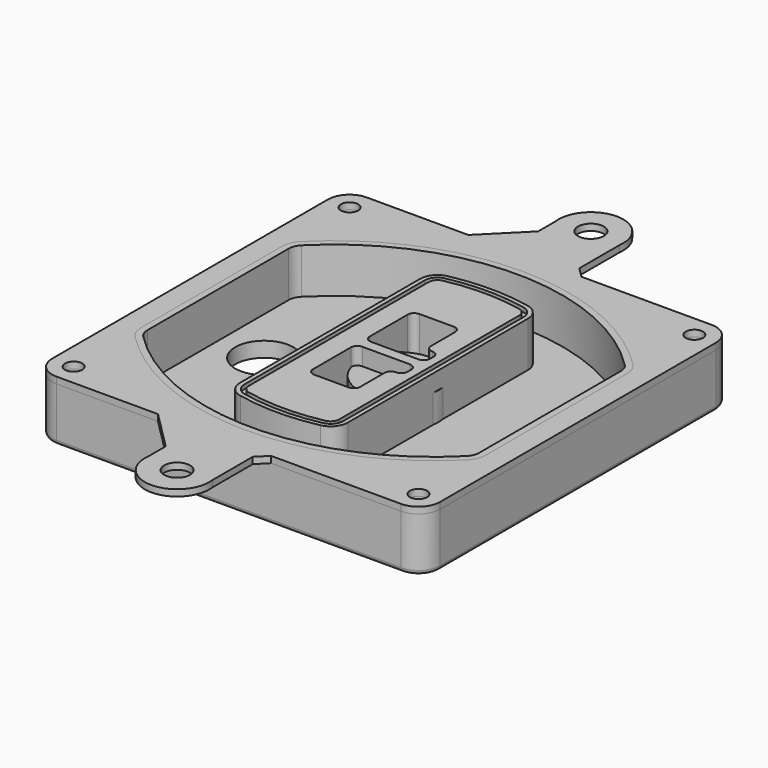
from build123d import *

# Parameters (mm, degrees)
F0_R      = 4
F1_DEPTH  = 25
F2_DEPTH  = 3
F3_DEPTH  = 18
F5_DEPTH  = 21
F6_DEPTH  = 2
F8_DEPTH  = 20
F9_DEPTH  = 16
F10_DEPTH = 25
F7_R      = 6
F7_R_2    = 4
F11_DEPTH = 6
F13_DEPTH = 9
F15_R     = 2
F16_R     = 6
F16_R_2   = 4
F17_DEPTH = 3


# Not quite as in the source:
# - a feature of the source that left no trace in its solid (it failed there, or was rolled back) is left out
# - a feature names something its author has since deleted; it is built from what else it names


with BuildPart() as f1:
    # F0 (on Top) → F1 (new body)
    with BuildSketch(Plane.XY):
        with BuildLine():
            ThreePointArc((-90, -80), (-87.0710678119, -87.0710678119), (-80, -90))
            Line((-80, -90), (80, -90))
            ThreePointArc((80, -90), (87.0710678119, -87.0710678119), (90, -80))
            Line((90, -80), (90, 80))
            ThreePointArc((90, 80), (87.0710678119, 87.0710678119), (80, 90))
            Line((80, 90), (-80, 90))
            ThreePointArc((-80, 90), (-87.0710678119, 87.0710678119), (-90, 80))
            Line((-90, 80), (-90, -80))
        make_face()
        with Locations((-80, -80)):
            Circle(F0_R, mode=Mode.SUBTRACT)
        with Locations((80, -80)):
            Circle(F0_R, mode=Mode.SUBTRACT)
        with Locations((-80, 80)):
            Circle(F0_R, mode=Mode.SUBTRACT)
        with BuildLine():
            ThreePointArc((-84, 40.977524478), (-82.9361107095, 46.3307515151), (-79.9061371841, 50.8703727074))
            ThreePointArc((-79.9061371841, 50.8703727074), (0, 84), (79.9061371841, 50.8703727074))
            ThreePointArc((79.9061371841, 50.8703727074), (82.9361107095, 46.3307515151), (84, 40.977524478))
            Line((84, 40.977524478), (84, -40.977524478))
            ThreePointArc((84, -40.977524478), (82.9361107095, -46.3307515151), (79.9061371841, -50.8703727074))
            ThreePointArc((79.9061371841, -50.8703727074), (0, -84), (-79.9061371841, -50.8703727074))
            ThreePointArc((-79.9061371841, -50.8703727074), (-82.9361107095, -46.3307515151), (-84, -40.977524478))
            Line((-84, -40.977524478), (-84, 40.977524478))
        make_face(mode=Mode.SUBTRACT)
        with Locations((80, 80)):
            Circle(F0_R, mode=Mode.SUBTRACT)
        with BuildLine():
            ThreePointArc((79.9061371841, 50.8703727074), (0, 84), (-79.9061371841, 50.8703727074))
            ThreePointArc((-79.9061371841, 50.8703727074), (-82.9361107095, 46.3307515151), (-84, 40.977524478))
            Line((-84, 40.977524478), (-84, -40.977524478))
            ThreePointArc((-84, -40.977524478), (-82.9361107095, -46.3307515151), (-79.9061371841, -50.8703727074))
            ThreePointArc((-79.9061371841, -50.8703727074), (0, -84), (79.9061371841, -50.8703727074))
            ThreePointArc((79.9061371841, -50.8703727074), (82.9361107095, -46.3307515151), (84, -40.977524478))
            Line((84, -40.977524478), (84, 40.977524478))
            ThreePointArc((84, 40.977524478), (82.9361107095, 46.3307515151), (79.9061371841, 50.8703727074))
        make_face()
        with BuildLine():
            Line((-80, -40.977524478), (-80, 40.977524478))
            ThreePointArc((-80, 40.977524478), (-79.2400790782, 44.801258076), (-77.0758122744, 48.0438446418))
            ThreePointArc((-77.0758122744, 48.0438446418), (0, 80), (77.0758122744, 48.0438446418))
            ThreePointArc((77.0758122744, 48.0438446418), (79.2400790782, 44.801258076), (80, 40.977524478))
            Line((80, 40.977524478), (80, -40.977524478))
            ThreePointArc((80, -40.977524478), (79.2400790782, -44.801258076), (77.0758122744, -48.0438446418))
            ThreePointArc((77.0758122744, -48.0438446418), (0, -80), (-77.0758122744, -48.0438446418))
            ThreePointArc((-77.0758122744, -48.0438446418), (-79.2400790782, -44.801258076), (-80, -40.977524478))
        make_face(mode=Mode.SUBTRACT)
        with BuildLine():
            ThreePointArc((-77.0758122744, 48.0438446418), (-79.2400790782, 44.801258076), (-80, 40.977524478))
            Line((-80, 40.977524478), (-80, -40.977524478))
            ThreePointArc((-80, -40.977524478), (-79.2400790782, -44.801258076), (-77.0758122744, -48.0438446418))
            ThreePointArc((-77.0758122744, -48.0438446418), (0, -80), (77.0758122744, -48.0438446418))
            ThreePointArc((77.0758122744, -48.0438446418), (79.2400790782, -44.801258076), (80, -40.977524478))
            Line((80, -40.977524478), (80, 40.977524478))
            ThreePointArc((80, 40.977524478), (79.2400790782, 44.801258076), (77.0758122744, 48.0438446418))
            ThreePointArc((77.0758122744, 48.0438446418), (0, 80), (-77.0758122744, 48.0438446418))
        make_face()
        with BuildLine():
            ThreePointArc((74.9530685921, 45.9239485927), (76.4680553548, 43.6541379966), (77, 40.977524478))
            Line((77, 40.977524478), (77, -40.977524478))
            ThreePointArc((77, -40.977524478), (76.4680553548, -43.6541379966), (74.9530685921, -45.9239485927))
            ThreePointArc((74.9530685921, -45.9239485927), (0, -77), (-74.9530685921, -45.9239485927))
            ThreePointArc((-74.9530685921, -45.9239485927), (-76.4680553548, -43.6541379966), (-77, -40.977524478))
            Line((-77, -40.977524478), (-77, 40.977524478))
            ThreePointArc((-77, 40.977524478), (-76.4680553548, 43.6541379966), (-74.9530685921, 45.9239485927))
            ThreePointArc((-74.9530685921, 45.9239485927), (0, 77), (74.9530685921, 45.9239485927))
        make_face(mode=Mode.SUBTRACT)
        with BuildLine():
            Line((77, -40.977524478), (77, 40.977524478))
            ThreePointArc((77, 40.977524478), (76.4680553548, 43.6541379966), (74.9530685921, 45.9239485927))
            ThreePointArc((74.9530685921, 45.9239485927), (0, 77), (-74.9530685921, 45.9239485927))
            ThreePointArc((-74.9530685921, 45.9239485927), (-76.4680553548, 43.6541379966), (-77, 40.977524478))
            Line((-77, 40.977524478), (-77, -40.977524478))
            ThreePointArc((-77, -40.977524478), (-76.4680553548, -43.6541379966), (-74.9530685921, -45.9239485927))
            ThreePointArc((-74.9530685921, -45.9239485927), (0, -77), (74.9530685921, -45.9239485927))
            ThreePointArc((74.9530685921, -45.9239485927), (76.4680553548, -43.6541379966), (77, -40.977524478))
        make_face()
    extrude(amount=-F1_DEPTH)

    # F0 (on Top) → F2 (join)
    with BuildSketch(Plane.XY):
        with BuildLine():
            ThreePointArc((-77.0758122744, 48.0438446418), (-79.2400790782, 44.801258076), (-80, 40.977524478))
            Line((-80, 40.977524478), (-80, -40.977524478))
            ThreePointArc((-80, -40.977524478), (-79.2400790782, -44.801258076), (-77.0758122744, -48.0438446418))
            ThreePointArc((-77.0758122744, -48.0438446418), (0, -80), (77.0758122744, -48.0438446418))
            ThreePointArc((77.0758122744, -48.0438446418), (79.2400790782, -44.801258076), (80, -40.977524478))
            Line((80, -40.977524478), (80, 40.977524478))
            ThreePointArc((80, 40.977524478), (79.2400790782, 44.801258076), (77.0758122744, 48.0438446418))
            ThreePointArc((77.0758122744, 48.0438446418), (0, 80), (-77.0758122744, 48.0438446418))
        make_face()
        with BuildLine():
            ThreePointArc((74.9530685921, 45.9239485927), (76.4680553548, 43.6541379966), (77, 40.977524478))
            Line((77, 40.977524478), (77, -40.977524478))
            ThreePointArc((77, -40.977524478), (76.4680553548, -43.6541379966), (74.9530685921, -45.9239485927))
            ThreePointArc((74.9530685921, -45.9239485927), (0, -77), (-74.9530685921, -45.9239485927))
            ThreePointArc((-74.9530685921, -45.9239485927), (-76.4680553548, -43.6541379966), (-77, -40.977524478))
            Line((-77, -40.977524478), (-77, 40.977524478))
            ThreePointArc((-77, 40.977524478), (-76.4680553548, 43.6541379966), (-74.9530685921, 45.9239485927))
            ThreePointArc((-74.9530685921, 45.9239485927), (0, 77), (74.9530685921, 45.9239485927))
        make_face(mode=Mode.SUBTRACT)
    extrude(amount=F2_DEPTH)

    # F0 (on Top) → F3 (cut)
    with BuildSketch(Plane.XY):
        with BuildLine():
            Line((77, -40.977524478), (77, 40.977524478))
            ThreePointArc((77, 40.977524478), (76.4680553548, 43.6541379966), (74.9530685921, 45.9239485927))
            ThreePointArc((74.9530685921, 45.9239485927), (0, 77), (-74.9530685921, 45.9239485927))
            ThreePointArc((-74.9530685921, 45.9239485927), (-76.4680553548, 43.6541379966), (-77, 40.977524478))
            Line((-77, 40.977524478), (-77, -40.977524478))
            ThreePointArc((-77, -40.977524478), (-76.4680553548, -43.6541379966), (-74.9530685921, -45.9239485927))
            ThreePointArc((-74.9530685921, -45.9239485927), (0, -77), (74.9530685921, -45.9239485927))
            ThreePointArc((74.9530685921, -45.9239485927), (76.4680553548, -43.6541379966), (77, -40.977524478))
        make_face()
    extrude(amount=-F3_DEPTH, mode=Mode.SUBTRACT)

    # F4 (on face) → F5 (join, through all)
    with BuildSketch(Plane.XY.offset(3)):
        with BuildLine():
            ThreePointArc((-25, -52.2388355719), (-23.2096587819, -57.2826573186), (-18.6399655469, -60.0689385728))
            ThreePointArc((-18.6399655469, -60.0689385728), (0, -62), (18.6399655469, -60.0689385728))
            ThreePointArc((18.6399655469, -60.0689385728), (23.2096587819, -57.2826573186), (25, -52.2388355719))
            Line((25, -52.2388355719), (25, 52.2388355719))
            ThreePointArc((25, 52.2388355719), (23.2096587819, 57.2826573186), (18.6399655469, 60.0689385728))
            ThreePointArc((18.6399655469, 60.0689385728), (0, 62), (-18.6399655469, 60.0689385728))
            ThreePointArc((-18.6399655469, 60.0689385728), (-23.2096587819, 57.2826573186), (-25, 52.2388355719))
            Line((-25, 52.2388355719), (-25, -52.2388355719))
        make_face()
        with BuildLine():
            ThreePointArc((18.2299741602, 58.1114128226), (21.6572440864, 56.0217018819), (23, 52.2388355719))
            Line((23, 52.2388355719), (23, -52.2388355719))
            ThreePointArc((23, -52.2388355719), (21.6572440864, -56.0217018819), (18.2299741602, -58.1114128226))
            ThreePointArc((18.2299741602, -58.1114128226), (0, -60), (-18.2299741602, -58.1114128226))
            ThreePointArc((-18.2299741602, -58.1114128226), (-21.6572440864, -56.0217018819), (-23, -52.2388355719))
            Line((-23, -52.2388355719), (-23, 52.2388355719))
            ThreePointArc((-23, 52.2388355719), (-21.6572440864, 56.0217018819), (-18.2299741602, 58.1114128226))
            ThreePointArc((-18.2299741602, 58.1114128226), (0, 60), (18.2299741602, 58.1114128226))
        make_face(mode=Mode.SUBTRACT)
        with BuildLine():
            Line((23, -52.2388355719), (23, 52.2388355719))
            ThreePointArc((23, 52.2388355719), (21.6572440864, 56.0217018819), (18.2299741602, 58.1114128226))
            ThreePointArc((18.2299741602, 58.1114128226), (0, 60), (-18.2299741602, 58.1114128226))
            ThreePointArc((-18.2299741602, 58.1114128226), (-21.6572440864, 56.0217018819), (-23, 52.2388355719))
            Line((-23, 52.2388355719), (-23, -52.2388355719))
            ThreePointArc((-23, -52.2388355719), (-21.6572440864, -56.0217018819), (-18.2299741602, -58.1114128226))
            ThreePointArc((-18.2299741602, -58.1114128226), (0, -60), (18.2299741602, -58.1114128226))
            ThreePointArc((18.2299741602, -58.1114128226), (21.6572440864, -56.0217018819), (23, -52.2388355719))
        make_face()
        with BuildLine():
            ThreePointArc((17.8199827735, 56.1538870724), (20.104829391, 54.7607464453), (21, 52.2388355719))
            Line((21, 52.2388355719), (21, -52.2388355719))
            ThreePointArc((21, -52.2388355719), (20.104829391, -54.7607464453), (17.8199827735, -56.1538870724))
            ThreePointArc((17.8199827735, -56.1538870724), (0, -58), (-17.8199827735, -56.1538870724))
            ThreePointArc((-17.8199827735, -56.1538870724), (-20.104829391, -54.7607464453), (-21, -52.2388355719))
            Line((-21, -52.2388355719), (-21, 52.2388355719))
            ThreePointArc((-21, 52.2388355719), (-20.104829391, 54.7607464453), (-17.8199827735, 56.1538870724))
            ThreePointArc((-17.8199827735, 56.1538870724), (0, 58), (17.8199827735, 56.1538870724))
        make_face(mode=Mode.SUBTRACT)
        with BuildLine():
            Line((21, -52.2388355719), (21, 52.2388355719))
            ThreePointArc((21, 52.2388355719), (20.104829391, 54.7607464453), (17.8199827735, 56.1538870724))
            ThreePointArc((17.8199827735, 56.1538870724), (0, 58), (-17.8199827735, 56.1538870724))
            ThreePointArc((-17.8199827735, 56.1538870724), (-20.104829391, 54.7607464453), (-21, 52.2388355719))
            Line((-21, 52.2388355719), (-21, -52.2388355719))
            ThreePointArc((-21, -52.2388355719), (-20.104829391, -54.7607464453), (-17.8199827735, -56.1538870724))
            ThreePointArc((-17.8199827735, -56.1538870724), (0, -58), (17.8199827735, -56.1538870724))
            ThreePointArc((17.8199827735, -56.1538870724), (20.104829391, -54.7607464453), (21, -52.2388355719))
        make_face()
        with BuildLine():
            Line((-8, -2.5), (14, -2.5))
            ThreePointArc((14, -2.5), (16.1213203436, -3.3786796564), (17, -5.5))
            Line((17, -5.5), (17, -7.5))
            ThreePointArc((17, -7.5), (16.1213203436, -9.6213203436), (14, -10.5))
            ThreePointArc((14, -10.5), (11.8786796564, -11.3786796564), (11, -13.5))
            Line((11, -13.5), (11, -27.5))
            ThreePointArc((11, -27.5), (10.1213203436, -29.6213203436), (8, -30.5))
            Line((8, -30.5), (-8, -30.5))
            ThreePointArc((-8, -30.5), (-10.1213203436, -29.6213203436), (-11, -27.5))
            Line((-11, -27.5), (-11, -5.5))
            ThreePointArc((-11, -5.5), (-10.1213203436, -3.3786796564), (-8, -2.5))
        make_face(mode=Mode.SUBTRACT)
        with BuildLine():
            ThreePointArc((-8, 2.5), (-10.1213203436, 3.3786796564), (-11, 5.5))
            Line((-11, 5.5), (-11, 27.5))
            ThreePointArc((-11, 27.5), (-10.1213203436, 29.6213203436), (-8, 30.5))
            Line((-8, 30.5), (8, 30.5))
            ThreePointArc((8, 30.5), (10.1213203436, 29.6213203436), (11, 27.5))
            Line((11, 27.5), (11, 13.5))
            ThreePointArc((11, 13.5), (11.8786796564, 11.3786796564), (14, 10.5))
            ThreePointArc((14, 10.5), (16.1213203436, 9.6213203436), (17, 7.5))
            Line((17, 7.5), (17, 5.5))
            ThreePointArc((17, 5.5), (16.1213203436, 3.3786796564), (14, 2.5))
            Line((14, 2.5), (-8, 2.5))
        make_face(mode=Mode.SUBTRACT)
    extrude(amount=-F5_DEPTH)

    # F4 (on face) → F6 (cut)
    with BuildSketch(Plane.XY.offset(3)):
        with BuildLine():
            Line((23, -52.2388355719), (23, 52.2388355719))
            ThreePointArc((23, 52.2388355719), (21.6572440864, 56.0217018819), (18.2299741602, 58.1114128226))
            ThreePointArc((18.2299741602, 58.1114128226), (0, 60), (-18.2299741602, 58.1114128226))
            ThreePointArc((-18.2299741602, 58.1114128226), (-21.6572440864, 56.0217018819), (-23, 52.2388355719))
            Line((-23, 52.2388355719), (-23, -52.2388355719))
            ThreePointArc((-23, -52.2388355719), (-21.6572440864, -56.0217018819), (-18.2299741602, -58.1114128226))
            ThreePointArc((-18.2299741602, -58.1114128226), (0, -60), (18.2299741602, -58.1114128226))
            ThreePointArc((18.2299741602, -58.1114128226), (21.6572440864, -56.0217018819), (23, -52.2388355719))
        make_face()
        with BuildLine():
            ThreePointArc((17.8199827735, 56.1538870724), (20.104829391, 54.7607464453), (21, 52.2388355719))
            Line((21, 52.2388355719), (21, -52.2388355719))
            ThreePointArc((21, -52.2388355719), (20.104829391, -54.7607464453), (17.8199827735, -56.1538870724))
            ThreePointArc((17.8199827735, -56.1538870724), (0, -58), (-17.8199827735, -56.1538870724))
            ThreePointArc((-17.8199827735, -56.1538870724), (-20.104829391, -54.7607464453), (-21, -52.2388355719))
            Line((-21, -52.2388355719), (-21, 52.2388355719))
            ThreePointArc((-21, 52.2388355719), (-20.104829391, 54.7607464453), (-17.8199827735, 56.1538870724))
            ThreePointArc((-17.8199827735, 56.1538870724), (0, 58), (17.8199827735, 56.1538870724))
        make_face(mode=Mode.SUBTRACT)
    extrude(amount=-F6_DEPTH, mode=Mode.SUBTRACT)

    # F7 (on face) → F8 (join)
    with BuildSketch(Plane(origin=(0, 0, -25), x_dir=(1, 0, 0), z_dir=(0, 0, -1))):
        with BuildLine():
            ThreePointArc((-6.71157564, 0), (6.7567035675, 13.4682792075), (20.224982775, 0))
            Line((20.224982775, 0), (25.224982775, 0))
            ThreePointArc((25.224982775, 0), (6.7567035675, 18.4682792075), (-11.71157564, 0))
            Line((-11.71157564, 0), (-6.71157564, 0))
        make_face()
        with BuildLine():
            Line((-6.71157564, 0), (20.224982775, 0))
            ThreePointArc((20.224982775, 0), (6.7567035675, 13.4682792075), (-6.71157564, 0))
        make_face()
        with BuildLine():
            ThreePointArc((-6.71157564, 0), (6.7567035675, -13.4682792075), (20.224982775, 0))
            Line((20.224982775, 0), (-6.71157564, 0))
        make_face()
        with BuildLine():
            Line((25.224982775, 0), (20.224982775, 0))
            ThreePointArc((20.224982775, 0), (6.7567035675, -13.4682792075), (-6.71157564, 0))
            Line((-6.71157564, 0), (-11.71157564, 0))
            ThreePointArc((-11.71157564, 0), (6.7567035675, -18.4682792075), (25.224982775, 0))
        make_face()
    extrude(amount=-F8_DEPTH)

    # F7 (on face) → F9 (cut)
    with BuildSketch(Plane(origin=(0, 0, -25), x_dir=(1, 0, 0), z_dir=(0, 0, -1))):
        with BuildLine():
            Line((-6.71157564, 0), (20.224982775, 0))
            ThreePointArc((20.224982775, 0), (6.7567035675, 13.4682792075), (-6.71157564, 0))
        make_face()
        with BuildLine():
            ThreePointArc((-6.71157564, 0), (6.7567035675, -13.4682792075), (20.224982775, 0))
            Line((20.224982775, 0), (-6.71157564, 0))
        make_face()
    extrude(amount=-F9_DEPTH, mode=Mode.SUBTRACT)

    # F7 (on face) → F10 (cut)
    with BuildSketch(Plane(origin=(0, 0, -25), x_dir=(1, 0, 0), z_dir=(0, 0, -1))):
        with BuildLine():
            Line((-69.0318229325, 0), (-42.0952645175, 0))
            ThreePointArc((-42.0952645175, 0), (-55.563543725, 13.4682792075), (-69.0318229325, 0))
        make_face()
        with BuildLine():
            ThreePointArc((-69.0318229325, 0), (-55.563543725, -13.4682792075), (-42.0952645175, 0))
            Line((-42.0952645175, 0), (-69.0318229325, 0))
        make_face()
    extrude(amount=-F10_DEPTH, mode=Mode.SUBTRACT)

    # F7 (on face) → F11 (cut)
    with BuildSketch(Plane(origin=(0, 0, -25), x_dir=(1, 0, 0), z_dir=(0, 0, -1))):
        with Locations((80, -80)):
            Circle(F7_R)
        with Locations((80, -80)):
            Circle(F7_R_2, mode=Mode.SUBTRACT)
        with Locations((-80, -80)):
            Circle(F7_R)
        with Locations((-80, -80)):
            Circle(F7_R_2, mode=Mode.SUBTRACT)
        with Locations((-80, 80)):
            Circle(F7_R)
        with Locations((-80, 80)):
            Circle(F7_R_2, mode=Mode.SUBTRACT)
        with Locations((80, 80)):
            Circle(F7_R)
        with Locations((80, 80)):
            Circle(F7_R_2, mode=Mode.SUBTRACT)
    extrude(amount=-F11_DEPTH, mode=Mode.SUBTRACT)

    # F12 (on face) → F13 (cut, through all)
    with BuildSketch(Plane(origin=(0, 0, -9), x_dir=(1, 0, 0), z_dir=(0, 0, -1))):
        with BuildLine():
            ThreePointArc((20.224982775, 0), (20.1663399806, 1.2554664788), (19.9909222755, 2.5))
            Line((19.9909222755, 2.5), (14, 2.5))
            ThreePointArc((14, 2.5), (16.1213203436, 3.3786796564), (17, 5.5))
            Line((17, 5.5), (17, 7.5))
            ThreePointArc((17, 7.5), (16.1213203436, 9.6213203436), (14, 10.5))
            ThreePointArc((14, 10.5), (12.1627255951, 11.1284134507), (11.0951631559, 12.750384826))
            ThreePointArc((11.0951631559, 12.750384826), (11.0476113807, 12.7664660322), (11, 12.7823698976))
            Line((11, 12.7823698976), (11, -12.7823698976))
            ThreePointArc((11, -12.7823698976), (11.0476113807, -12.7664660322), (11.0951631559, -12.750384826))
            ThreePointArc((11.0951631559, -12.750384826), (12.1627255951, -11.1284134507), (14, -10.5))
            ThreePointArc((14, -10.5), (16.1213203436, -9.6213203436), (17, -7.5))
            Line((17, -7.5), (17, -5.5))
            ThreePointArc((17, -5.5), (16.1213203436, -3.3786796564), (14, -2.5))
            Line((14, -2.5), (19.9909222755, -2.5))
            ThreePointArc((19.9909222755, -2.5), (20.1663399806, -1.2554664788), (20.224982775, 0))
        make_face()
    extrude(amount=F13_DEPTH, mode=Mode.SUBTRACT)

    # F15
    f15_edges = [f1.edges().sort_by_distance(p)[0] for p in [
        (0, -90, -25),
        (-87.071068, -87.071068, -25),
        (-90, 0, -25),
        (-87.071068, 87.071068, -25),
        (87.071068, -87.071068, -25),
        (0, 90, -25),
        (90, 0, -25),
        (87.071068, 87.071068, -25),
    ]]
    fillet(f15_edges, radius=F15_R)


with BuildPart() as f17:
    # F16 (on face) → F17 (new body, through all)
    with BuildSketch(Plane.XY):
        with BuildLine():
            Line((19.5972977877, -90), (-32.8713560282, -90))
            Line((-32.8713560282, -90), (-14.8713560282, -108))
            Line((-14.8713560282, -108), (-14.8713560282, -118.0397015834))
            ThreePointArc((-14.8713560282, -118.0397015834), (0, -135), (14.8713560282, -118.0397015834))
            Line((14.8713560282, -118.0397015834), (14.8713560282, -94.7259417595))
            Line((14.8713560282, -94.7259417595), (19.5972977877, -90))
        make_face()
        with Locations((0, -120)):
            Circle(F16_R, mode=Mode.SUBTRACT)
        with BuildLine():
            Line((-14.8713560282, 118.0397015834), (-14.8713560282, 108))
            Line((-14.8713560282, 108), (-32.8713560282, 90))
            Line((-32.8713560282, 90), (19.5972977877, 90))
            Line((19.5972977877, 90), (14.8713560282, 94.7259417595))
            Line((14.8713560282, 94.7259417595), (14.8713560282, 118.0397015834))
            ThreePointArc((14.8713560282, 118.0397015834), (0, 135), (-14.8713560282, 118.0397015834))
        make_face()
        with Locations((0, 120)):
            Circle(F16_R, mode=Mode.SUBTRACT)
        with BuildLine():
            Line((19.5972977877, 90), (-32.8713560282, 90))
            Line((-32.8713560282, 90), (-80, 90))
            ThreePointArc((-80, 90), (-87.0710678119, 87.0710678119), (-90, 80))
            Line((-90, 80), (-90, -80))
            ThreePointArc((-90, -80), (-87.0710678119, -87.0710678119), (-80, -90))
            Line((-80, -90), (-32.8713560282, -90))
            Line((-32.8713560282, -90), (19.5972977877, -90))
            Line((19.5972977877, -90), (80, -90))
            ThreePointArc((80, -90), (87.0710678119, -87.0710678119), (90, -80))
            Line((90, -80), (90, 80))
            ThreePointArc((90, 80), (87.0710678119, 87.0710678119), (80, 90))
            Line((80, 90), (19.5972977877, 90))
        make_face()
        with Locations((-80, -80)):
            Circle(F16_R_2, mode=Mode.SUBTRACT)
        with Locations((80, -80)):
            Circle(F16_R_2, mode=Mode.SUBTRACT)
        with BuildLine():
            ThreePointArc((-80, 40.977524478), (-79.2400790782, 44.801258076), (-77.0758122744, 48.0438446418))
            ThreePointArc((-77.0758122744, 48.0438446418), (0, 80), (77.0758122744, 48.0438446418))
            ThreePointArc((77.0758122744, 48.0438446418), (79.2400790782, 44.801258076), (80, 40.977524478))
            Line((80, 40.977524478), (80, -40.977524478))
            ThreePointArc((80, -40.977524478), (79.2400790782, -44.801258076), (77.0758122744, -48.0438446418))
            ThreePointArc((77.0758122744, -48.0438446418), (0, -80), (-77.0758122744, -48.0438446418))
            ThreePointArc((-77.0758122744, -48.0438446418), (-79.2400790782, -44.801258076), (-80, -40.977524478))
            Line((-80, -40.977524478), (-80, 40.977524478))
        make_face(mode=Mode.SUBTRACT)
        with Locations((-80, 80)):
            Circle(F16_R_2, mode=Mode.SUBTRACT)
        with Locations((80, 80)):
            Circle(F16_R_2, mode=Mode.SUBTRACT)
    extrude(amount=F17_DEPTH)


solid = Compound([f1.part, f17.part])
